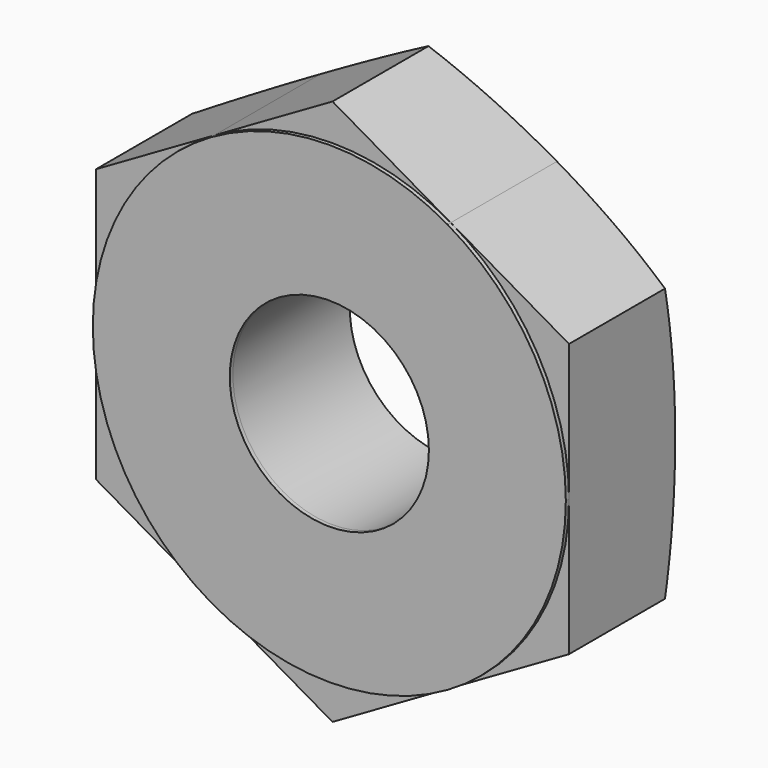
from build123d import *

# Parameters (mm, degrees)
F0_R        = 3.175
F1_DEPTH    = 5.08
F4_DEPTH    = 0.127
F5_T2_ANGLE = 270.0000002743
F5_T4_ANGLE = 89.9999990242


# Not quite as in the source:
# - a fillet or chamfer that OpenCascade refuses, or shapes differently, is made with other operations: its cross-section is extruded or revolved along the edge and cut away or added


with BuildPart() as f1:
    # F0 (on Front) → F1 (new body)
    with BuildSketch(Plane.XZ):
        with BuildLine():
            ThreePointArc((3.7703126428, -6.530372728), (6.5303728516, -3.7703124286), (7.540625, 0))
            ThreePointArc((7.540625, 0), (6.53037284, 3.7703124487), (3.7703126026, 6.5303727512))
            ThreePointArc((3.7703126026, 6.5303727512), (1.138e-07, 7.540625), (-3.7703124055, 6.530372865))
            ThreePointArc((-3.7703124055, 6.530372865), (-6.5303727831, 3.7703125473), (-7.540625, 0))
            ThreePointArc((-7.540625, 0), (-6.5303727946, -3.7703125273), (-3.7703124454, -6.5303728419))
            ThreePointArc((-3.7703124454, -6.5303728419), (1.14e-07, -7.540625), (3.7703126428, -6.530372728))
        make_face()
        Circle(F0_R, mode=Mode.SUBTRACT)
        with BuildLine():
            ThreePointArc((-3.7703124055, 6.530372865), (1.138e-07, 7.540625), (3.7703126026, 6.5303727512))
            Line((3.7703126026, 6.5303727512), (0, 8.7071637472))
            Line((0, 8.7071637472), (-3.7703124055, 6.530372865))
        make_face()
        with BuildLine():
            ThreePointArc((3.7703126026, 6.5303727512), (6.53037284, 3.7703124487), (7.540625, 0))
            Line((7.540625, 0), (7.540625, 4.3535818736))
            Line((7.540625, 4.3535818736), (3.7703126026, 6.5303727512))
        make_face()
        with BuildLine():
            Line((7.540625, -4.3535818736), (7.540625, 0))
            ThreePointArc((7.540625, 0), (6.5303728516, -3.7703124286), (3.7703126428, -6.530372728))
            Line((3.7703126428, -6.530372728), (7.540625, -4.3535818736))
        make_face()
        with BuildLine():
            Line((0, -8.7071637472), (3.7703126428, -6.530372728))
            ThreePointArc((3.7703126428, -6.530372728), (1.14e-07, -7.540625), (-3.7703124454, -6.5303728419))
            Line((-3.7703124454, -6.5303728419), (0, -8.7071637472))
        make_face()
        with BuildLine():
            Line((-7.540625, -4.3535818736), (-3.7703124454, -6.5303728419))
            ThreePointArc((-3.7703124454, -6.5303728419), (-6.5303727946, -3.7703125273), (-7.540625, 0))
            Line((-7.540625, 0), (-7.540625, -4.3535818736))
        make_face()
        with BuildLine():
            ThreePointArc((-7.540625, 0), (-6.5303727831, 3.7703125473), (-3.7703124055, 6.530372865))
            Line((-3.7703124055, 6.530372865), (-7.540625, 4.3535818736))
            Line((-7.540625, 4.3535818736), (-7.540625, 0))
        make_face()
    extrude(amount=-F1_DEPTH)

    # F2 (on Right) → F3 (revolve, cut)
    with BuildSketch(Plane.YZ):
        with BuildLine():
            Line((3.81, 9.0924566612), (3.81, 8.7445406243))
            add(Edge.make_bspline(
                [(3.81, 8.7445406243), (5.3219394758, 4.8979949206), (5.10083884, 1.2277201749), (5.1008383743, 0)],
                knots=[0, 0, 0, 0, 8.8393016941, 8.8393016941, 8.8393016941, 8.8393016941], degree=3))
            Line((5.1008383743, 0), (5.7132975198, 0))
            Line((5.7132975198, 0), (5.843443796, 9.0924566612))
            Line((5.843443796, 9.0924566612), (3.81, 9.0924566612))
        make_face()
    revolve(axis=Axis((0, 3.8655868266, 0), (0, 1, 0)), mode=Mode.SUBTRACT)

    # F0 (on Front) → F4 (join)
    with BuildSketch(Plane.XZ):
        with BuildLine():
            ThreePointArc((3.7703126428, -6.530372728), (6.5303728516, -3.7703124286), (7.540625, 0))
            ThreePointArc((7.540625, 0), (6.53037284, 3.7703124487), (3.7703126026, 6.5303727512))
            ThreePointArc((3.7703126026, 6.5303727512), (1.138e-07, 7.540625), (-3.7703124055, 6.530372865))
            ThreePointArc((-3.7703124055, 6.530372865), (-6.5303727831, 3.7703125473), (-7.540625, 0))
            ThreePointArc((-7.540625, 0), (-6.5303727946, -3.7703125273), (-3.7703124454, -6.5303728419))
            ThreePointArc((-3.7703124454, -6.5303728419), (1.14e-07, -7.540625), (3.7703126428, -6.530372728))
        make_face()
        Circle(F0_R, mode=Mode.SUBTRACT)
    extrude(amount=F4_DEPTH)

    # F5: chamfer of 0.381 on 2 edges, made by hand

    # F5_s1 → F5_t2 (revolve, cut)
    with BuildSketch(Plane.YZ.offset(-2.52e-08)):
        with BuildLine():
            Line((5.0173010484, 3.5721368448), (4.6454183479, 3.163731628))
            Line((4.6454183479, 3.163731628), (4.6454183479, 3.156111628))
            ThreePointArc((4.6454183479, 3.156111628), (4.8426673099, 3.1673799993), (5.039916272, 3.16738))
            Line((5.039916272, 3.16738), (5.0475139696, 3.1755825719))
            ThreePointArc((5.0475139696, 3.1755825719), (5.0314515178, 3.3738112251), (5.0248877329, 3.5728486159))
            Line((5.0248877329, 3.5728486159), (5.0173010484, 3.5721368448))
        make_face()
    revolve(axis=Axis((-2.52e-08, 5.039916272, 1e-08), (0, -1, 0)), revolution_arc=F5_T2_ANGLE, mode=Mode.SUBTRACT)

    # F5_s3 → F5_t4 (revolve, cut)
    with BuildSketch(Plane.XY.offset(-1.33e-08)):
        with BuildLine():
            Line((3.572136843, 5.0173010484), (3.1637316262, 4.6454183479))
            Line((3.1637316262, 4.6454183479), (3.1561116262, 4.6454183479))
            ThreePointArc((3.1561116262, 4.6454183479), (3.1673799975, 4.84266731), (3.16738, 5.039916272))
            Line((3.16738, 5.039916272), (3.1755825719, 5.0475139696))
            ThreePointArc((3.1755825719, 5.0475139696), (3.3738112242, 5.0314515177), (3.572848614, 5.0248877329))
            Line((3.572848614, 5.0248877329), (3.572136843, 5.0173010484))
        make_face()
    revolve(axis=Axis((-4.08e-08, 5.039916272, -1.33e-08), (0, -1, 0)), revolution_arc=F5_T4_ANGLE, mode=Mode.SUBTRACT)


solid = f1.part
